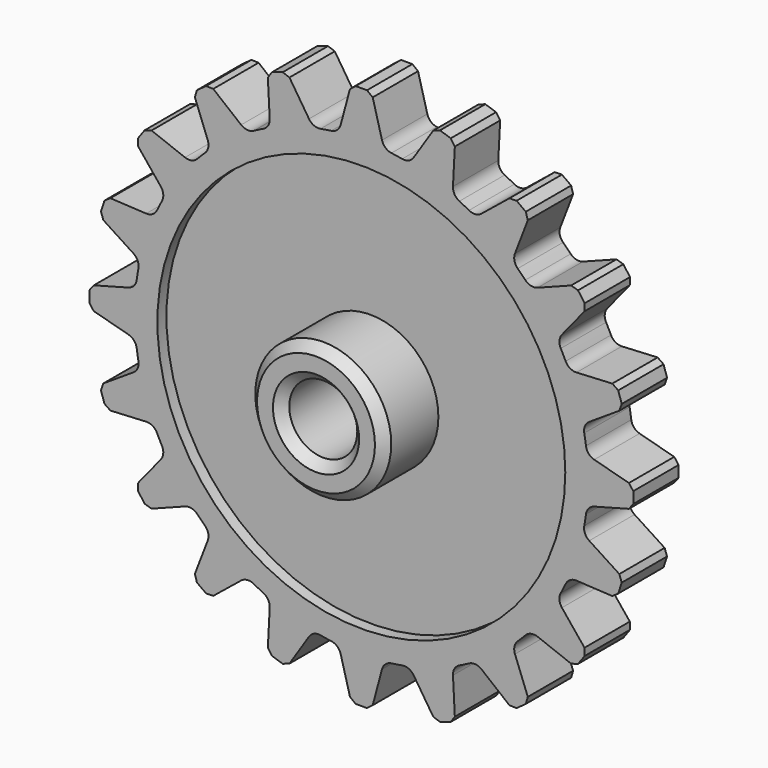
from build123d import *

# Parameters (mm, degrees)
F0_R            = 100
F1_DEPTH        = 25
F3_DEPTH        = 25
F3_COPIES_COUNT = 20
F4_SIZE         = 2
F5_R            = 5
F6_R            = 90
F7_DEPTH        = 5
F8_R            = 30
F9_DEPTH        = 30
F10_R           = 15
F11_DEPTH       = 50.001
F12_SIZE        = 4


# Not quite as in the source:
# - a pattern or mirror of a feature is missing from the dataset's text; its kind, count and spacing are read off the source's solid


with BuildPart() as f1:
    # F0 (on Front) → F1 (new body)
    with BuildSketch(Plane.XZ):
        Circle(F0_R)
    extrude(amount=F1_DEPTH)

    # F2 (on Front) → F3 (join)
    with BuildSketch(Plane.XZ):
        Polygon((-4.5, 120), (-9.9931095726, 99.4994359837), (9.9931095726, 99.4994359837), (4.5, 120), align=None)
    f3 = extrude(amount=F3_DEPTH)

    # F3_copies: F3 ×20 about axis
    f3_copies_axis = Axis((0, 0, 0), (0, 1, 0))
    for i in range(1, F3_COPIES_COUNT):
        add(f3.rotate(f3_copies_axis, i * 360 / F3_COPIES_COUNT))

    # F4
    f4_edges = [f1.edges().sort_by_distance(p)[0] for p in [
        (4.5, -12.5, 120),
        (-4.5, -12.5, 120),
        (-32.802285, -12.5, 115.517358),
        (115.517358, -12.5, 32.802285),
        (120, -12.5, 4.5),
        (120, -12.5, -4.5),
        (115.517358, -12.5, -32.802285),
        (112.736205, -12.5, -41.361794),
        (99.727073, -12.5, -66.893654),
        (94.437006, -12.5, -74.174807),
        (74.174807, -12.5, -94.437006),
        (66.893654, -12.5, -99.727073),
        (41.361794, -12.5, -112.736205),
        (32.802285, -12.5, -115.517358),
        (4.5, -12.5, -120),
        (-4.5, -12.5, -120),
        (-32.802285, -12.5, -115.517358),
        (-41.361794, -12.5, -112.736205),
        (-66.893654, -12.5, -99.727073),
        (-74.174807, -12.5, -94.437006),
        (-94.437006, -12.5, -74.174807),
        (-99.727073, -12.5, -66.893654),
        (-112.736205, -12.5, -41.361794),
        (-115.517358, -12.5, -32.802285),
        (-120, -12.5, -4.5),
        (-120, -12.5, 4.5),
        (-115.517358, -12.5, 32.802285),
        (-112.736205, -12.5, 41.361794),
        (-99.727073, -12.5, 66.893654),
        (-94.437006, -12.5, 74.174807),
        (-74.174807, -12.5, 94.437006),
        (-66.893654, -12.5, 99.727073),
        (32.802285, -12.5, 115.517358),
        (41.361794, -12.5, 112.736205),
        (66.893654, -12.5, 99.727073),
        (74.174807, -12.5, 94.437006),
        (94.437006, -12.5, 74.174807),
        (99.727073, -12.5, 66.893654),
        (112.736205, -12.5, 41.361794),
        (-41.361794, -12.5, 112.736205),
    ]]
    chamfer(f4_edges, length=F4_SIZE)

    # F5
    f5_edges = [f1.edges().sort_by_distance(p)[0] for p in [
        (9.99311, -12.5, 99.499436),
        (-9.99311, -12.5, 99.499436),
        (97.717628, -12.5, 21.243005),
        (99.499436, -12.5, 9.99311),
        (91.541546, -12.5, 40.251029),
        (86.370537, -12.5, 50.399706),
        (99.499436, -12.5, -9.99311),
        (97.717628, -12.5, -21.243005),
        (74.622932, -12.5, 66.568897),
        (66.568897, -12.5, 74.622932),
        (91.541546, -12.5, -40.251029),
        (86.370537, -12.5, -50.399706),
        (50.399706, -12.5, 86.370537),
        (40.251029, -12.5, 91.541546),
        (74.622932, -12.5, -66.568897),
        (66.568897, -12.5, -74.622932),
        (21.243005, -12.5, 97.717628),
        (50.399706, -12.5, -86.370537),
        (40.251029, -12.5, -91.541546),
        (-21.243005, -12.5, 97.717628),
        (21.243005, -12.5, -97.717628),
        (9.99311, -12.5, -99.499436),
        (-40.251029, -12.5, 91.541546),
        (-50.399706, -12.5, 86.370537),
        (-9.99311, -12.5, -99.499436),
        (-21.243005, -12.5, -97.717628),
        (-66.568897, -12.5, 74.622932),
        (-74.622932, -12.5, 66.568897),
        (-40.251029, -12.5, -91.541546),
        (-50.399706, -12.5, -86.370537),
        (-86.370537, -12.5, 50.399706),
        (-91.541546, -12.5, 40.251029),
        (-66.568897, -12.5, -74.622932),
        (-74.622932, -12.5, -66.568897),
        (-97.717628, -12.5, 21.243005),
        (-99.499436, -12.5, 9.99311),
        (-86.370537, -12.5, -50.399706),
        (-91.541546, -12.5, -40.251029),
        (-99.499436, -12.5, -9.99311),
        (-97.717628, -12.5, -21.243005),
    ]]
    fillet(f5_edges, radius=F5_R)

    # F6 (on face) → F7 (cut)
    with BuildSketch(Plane.XZ.offset(25)):
        Circle(F6_R)
    extrude(amount=-F7_DEPTH, mode=Mode.SUBTRACT)

    # F8 (on face) → F9 (join)
    with BuildSketch(Plane.XZ.offset(20)):
        Circle(F8_R)
    extrude(amount=F9_DEPTH)

    # F10 (on face) → F11 (cut, through all)
    with BuildSketch(Plane.XZ.offset(50)):
        Circle(F10_R)
    extrude(amount=-F11_DEPTH, mode=Mode.SUBTRACT)

    # F12
    f12_edges = [f1.edges().sort_by_distance(p)[0] for p in [
        (-30, -50, 0),
        (-15, -50, 0),
    ]]
    chamfer(f12_edges, length=F12_SIZE)


solid = f1.part
